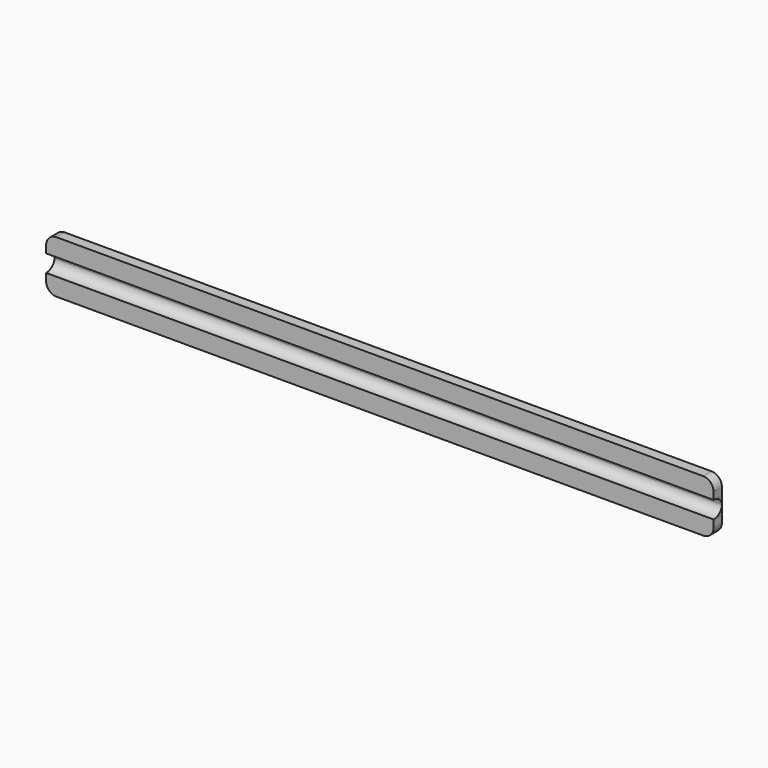
from build123d import *

# Parameters (mm, degrees)
F0_W     = 203.2
F0_H     = 5.355444
F1_DEPTH = 3.175
F2_DEPTH = 3.175
F4_DEPTH = 203.2
F5_R     = 3.175
F5_2_R   = 3.175


with BuildPart() as f1:
    # F0 (on Front) → F1 (new body)
    with BuildSketch(Plane.XZ):
        with Locations((3.755528, 5.751835)):
            Rectangle(F0_W, F0_H)
    extrude(amount=F1_DEPTH)

    # F5
    f5_edges = [f1.edges().sort_by_distance(p)[0] for p in [
        (-97.844472, -1.5875, 8.429557),
        (105.355528, -1.5875, 8.429557),
    ]]
    fillet(f5_edges, radius=F5_R)


with BuildPart() as f1b:
    # F0 (on Front) → F1, piece 2 (new body)
    with BuildSketch(Plane.XZ):
        with Locations((3.755528, -4.83585)):
            Rectangle(F0_W, F0_H)
    extrude(amount=F1_DEPTH)

    # F5#2
    f5_2_edges = [f1b.edges().sort_by_distance(p)[0] for p in [
        (-97.844472, -1.5875, -7.513572),
        (105.355528, -1.5875, -7.513572),
    ]]
    fillet(f5_2_edges, radius=F5_2_R)


with BuildPart() as f2:
    # F0 (on Front) → F2 (new body)
    with BuildSketch(Plane.XZ):
        Polygon((105.355528, 3.074113), (-97.844472, 3.074113), (-97.844472, 0.457992), (-97.844472, -2.158128), (105.355528, -2.158128), (105.355528, 0.457992), align=None)
    extrude(amount=F2_DEPTH)

    # F3 (on face) → F4 (cut)
    with BuildSketch(Plane(origin=(-97.844472, 0, 0), x_dir=(0, -1, 0), z_dir=(-1, 0, 0))):
        with BuildLine():
            Line((3.175, -2.158128), (3.175, 3.074113))
            add(Edge.make_bspline(
                [(3.175, 3.074113), (1.279306, 3.074113), (0, 1.766053), (0, 0.457992)],
                knots=[0, 0, 0, 0, 0.5, 0.5, 0.5, 0.5], degree=3))
            add(Edge.make_bspline(
                [(0, 0.457992), (0, -0.850068), (1.279306, -2.158128), (3.175, -2.158128)],
                knots=[0.5, 0.5, 0.5, 0.5, 1, 1, 1, 1], degree=3))
        make_face()
    extrude(amount=-F4_DEPTH, mode=Mode.SUBTRACT)


solid = Compound([f1.part, f1b.part, f2.part])
